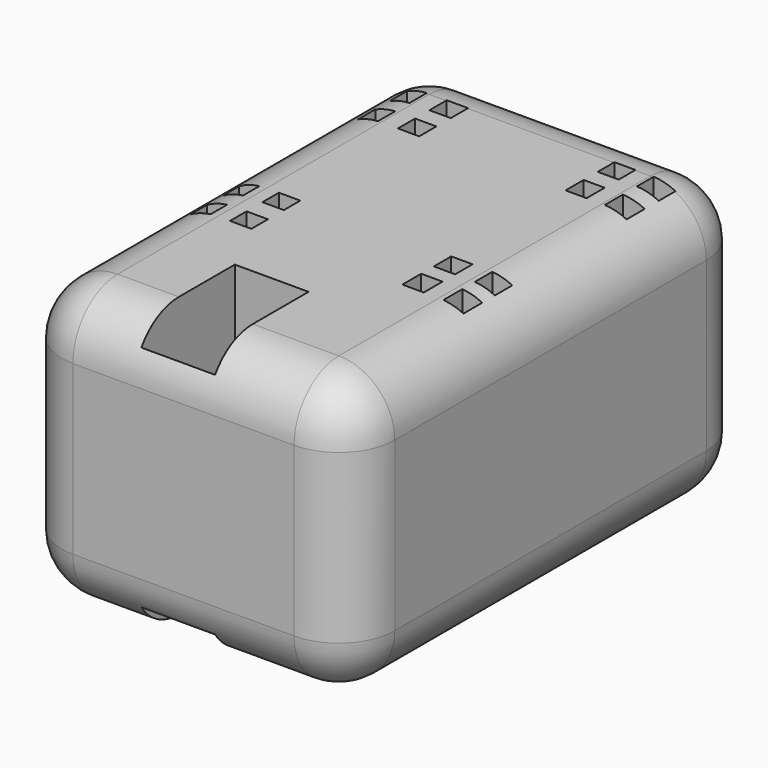
from build123d import *

# Parameters (mm, degrees)
F0_W         = 6.5923197919
F0_H         = 0.8001455572
F0_W_2       = 1.763837412
F0_H_2       = 1.412447542
F0_H_3       = 2.101770214
F0_W_3       = 1.9069323985
F0_H_4       = 1.9450464989
F0_W_4       = 1.7884944444
F0_W_5       = 1.6274210066
F0_H_5       = 1.5719905496
F0_H_6       = 1.8685259757
F0_W_6       = 1.9532360649
F0_H_7       = 2.0187458968
F0_W_7       = 1.8786090163
F0_W_8       = 1.7776318862
F0_H_8       = 1.6108304262
F0_W_9       = 1.7758645117
F0_H_9       = 1.9326903758
F0_H_10      = 1.91574162
F0_W_10      = 1.905767857
F0_W_11      = 1.7302669585
F0_H_11      = 1.8497077592
F0_H_12      = 1.7764922231
F0_H_13      = 1.8330642725
F0_W_12      = 1.8128681632
F0_W_13      = 1.9161291332
F1_DEPTH     = 25
F2_T1_DEPTH  = 34.8057161443
F2_T3_DEPTH  = 15
F2_T5_DEPTH  = 19.7681800186
F2_S9_W      = 5
F2_S9_H      = 5
F2_T10_DEPTH = 5
F2_S15_W     = 5
F2_S15_H     = 5
F2_T16_DEPTH = 5
F2_S21_W     = 5
F2_S21_H     = 5
F2_T22_DEPTH = 5
F2_S27_W     = 5
F2_S27_H     = 5
F2_T28_DEPTH = 5
F2_S33_W     = 5
F2_S33_H     = 5
F2_T34_DEPTH = 5
F2_S39_W     = 5
F2_S39_H     = 5
F2_T40_DEPTH = 5
F2_S45_W     = 5
F2_S45_H     = 5
F2_T46_DEPTH = 5
F2_S51_W     = 5
F2_S51_H     = 5
F2_T52_DEPTH = 5


# Not quite as in the source:
# - a fillet or chamfer that OpenCascade refuses, or shapes differently, is made with other operations: its cross-section is extruded or revolved along the edge and cut away or added


with BuildPart() as f1:
    # F0 (on Top) → F1 (new body)
    with BuildSketch(Plane.XY):
        with Locations((-41.465645377, 0.4000727786)):
            Rectangle(F0_W, F0_H)
        Polygon((-25.4717437439, 44.8057161443), (-55.2399237625, 44.8057161443), (-55.2399237625, 0), (-44.761805273, 0), (-44.761805273, 0.8001455572), (-44.761805273, 11.2422176864), (-38.1694854811, 11.2422176864), (-38.1694854811, 0.8001455572), (-38.1694854811, 0), (-25.4717437439, 0), (-25.4717437439, 44.1919353443), align=None)
        Polygon((-52.6931885334, 19.8126584291), (-52.6931885334, 21.6457227017), (-50.8803203702, 21.6457227017), (-49.1500534117, 21.6457227017), (-47.2339242785, 21.6457227017), (-47.2339242785, 19.8126584291), (-47.2339242785, 18.036166206), (-47.2339242785, 16.1864584468), (-49.1500534117, 16.1864584468), (-50.8803203702, 16.1864584468), (-52.6931885334, 16.1864584468), (-52.6931885334, 18.036166206), align=None, mode=Mode.SUBTRACT)
        Polygon((-30.0695020705, 21.6457227017), (-28.2810076261, 21.6457227017), (-28.2810076261, 19.7006762028), (-28.2810076261, 18.2882286608), (-28.2810076261, 16.1864584468), (-30.0695020705, 16.1864584468), (-31.8333394825, 16.1864584468), (-33.740271881, 16.1864584468), (-33.740271881, 18.2882286608), (-33.740271881, 19.7006762028), (-33.740271881, 21.6457227017), (-31.8333394825, 21.6457227017), align=None, mode=Mode.SUBTRACT)
        Polygon((-52.2811726703, 37.9449166358), (-52.2811726703, 39.8776070116), (-50.5035407841, 39.8776070116), (-48.7276762724, 39.8776070116), (-46.8219084154, 39.8776070116), (-46.8219084154, 37.9449166358), (-46.8219084154, 36.3340862095), (-46.8219084154, 34.4183445895), (-48.7276762724, 34.4183445895), (-50.5035407841, 34.4183445895), (-52.2811726703, 34.4183445895), (-52.2811726703, 36.3340862095), align=None, mode=Mode.SUBTRACT)
        Polygon((-30.2342418581, 39.8776070116), (-28.2810057933, 39.8776070116), (-28.2810057933, 38.0090810359), (-28.2810057933, 36.4370904863), (-28.2810057933, 34.4183445895), (-30.2342418581, 34.4183445895), (-31.8616628647, 34.4183445895), (-33.740271881, 34.4183445895), (-33.740271881, 36.4370904863), (-33.740271881, 38.0090810359), (-33.740271881, 39.8776070116), (-31.8616628647, 39.8776070116), align=None, mode=Mode.SUBTRACT)
        with Locations((-30.9514207765, 18.9944524318)):
            Rectangle(F0_W_2, F0_H_2)
        with Locations((-30.9514207765, 17.2373435538)):
            Rectangle(F0_W_2, F0_H_3)
        with Locations((-32.7868056818, 18.9944524318)):
            Rectangle(F0_W_3, F0_H_2)
        with Locations((-30.9514207765, 20.6731994522)):
            Rectangle(F0_W_2, F0_H_4)
        with Locations((-29.1752548483, 18.9944524318)):
            Rectangle(F0_W_4, F0_H_2)
        with Locations((-31.0479523614, 37.2230857611)):
            Rectangle(F0_W_5, F0_H_5)
        with Locations((-31.0479523614, 38.9433440237)):
            Rectangle(F0_W_5, F0_H_6)
        with Locations((-29.2576238257, 37.2230857611)):
            Rectangle(F0_W_6, F0_H_5)
        with Locations((-31.0479523614, 35.4277175379)):
            Rectangle(F0_W_5, F0_H_7)
        with Locations((-32.8009673728, 37.2230857611)):
            Rectangle(F0_W_7, F0_H_5)
        with Locations((-51.3923567272, 37.1395014226)):
            Rectangle(F0_W_8, F0_H_8)
        with Locations((-49.6156085283, 37.1395014226)):
            Rectangle(F0_W_9, F0_H_8)
        with Locations((-49.6156085283, 38.9112618237)):
            Rectangle(F0_W_9, F0_H_9)
        with Locations((-49.6156085283, 35.3762153995)):
            Rectangle(F0_W_9, F0_H_10)
        with Locations((-47.7747923439, 37.1395014226)):
            Rectangle(F0_W_10, F0_H_8)
        with Locations((-50.015186891, 17.1113123264)):
            Rectangle(F0_W_11, F0_H_11)
        with Locations((-50.015186891, 18.9244123176)):
            Rectangle(F0_W_11, F0_H_12)
        with Locations((-50.015186891, 20.7291905654)):
            Rectangle(F0_W_11, F0_H_13)
        with Locations((-51.7867544518, 18.9244123176)):
            Rectangle(F0_W_12, F0_H_12)
        with Locations((-48.1919888451, 18.9244123176)):
            Rectangle(F0_W_13, F0_H_12)
    extrude(amount=F1_DEPTH)

    # F2: fillet of radius 5 on 12 edges, made by hand

    # F2_s2 → F2_t1 (cut)
    with BuildSketch(Plane.XZ.offset(-39.8057161443)):
        with BuildLine():
            ThreePointArc((-25.4717437439, 5), (-26.9362098379, 1.4644660941), (-30.4717437439, 0))
            Line((-30.4717437439, 0), (-25.4717437439, 0))
            Line((-25.4717437439, 0), (-25.4717437439, 5))
        make_face()
        with BuildLine():
            ThreePointArc((-25.4717437439, 20), (-26.9362098379, 23.5355339059), (-30.4717437439, 25))
            Line((-30.4717437439, 25), (-25.4717437439, 25))
            Line((-25.4717437439, 25), (-25.4717437439, 20))
        make_face()
        with BuildLine():
            ThreePointArc((-55.2399237625, 5), (-53.7754576684, 1.4644660941), (-50.2399237625, 0))
            Line((-50.2399237625, 0), (-55.2399237625, 0))
            Line((-55.2399237625, 0), (-55.2399237625, 5))
        make_face()
        with BuildLine():
            ThreePointArc((-55.2399237625, 20), (-53.7754576684, 23.5355339059), (-50.2399237625, 25))
            Line((-50.2399237625, 25), (-55.2399237625, 25))
            Line((-55.2399237625, 25), (-55.2399237625, 20))
        make_face()
    extrude(amount=F2_T1_DEPTH, mode=Mode.SUBTRACT)

    # F2_s4 → F2_t3 (cut)
    with BuildSketch(Plane.XY.offset(5)):
        with BuildLine():
            ThreePointArc((-25.4717437439, 39.8057161443), (-26.9362098379, 43.3412500502), (-30.4717437439, 44.8057161443))
            Line((-30.4717437439, 44.8057161443), (-25.4717437439, 44.8057161443))
            Line((-25.4717437439, 44.8057161443), (-25.4717437439, 39.8057161443))
        make_face()
        with BuildLine():
            ThreePointArc((-50.2399237625, 44.8057161443), (-53.7754576684, 43.3412500502), (-55.2399237625, 39.8057161443))
            Line((-55.2399237625, 39.8057161443), (-55.2399237625, 44.8057161443))
            Line((-55.2399237625, 44.8057161443), (-50.2399237625, 44.8057161443))
        make_face()
        with BuildLine():
            ThreePointArc((-55.2399237625, 5), (-53.7754576684, 1.4644660941), (-50.2399237625, 0))
            Line((-50.2399237625, 0), (-55.2399237625, 0))
            Line((-55.2399237625, 0), (-55.2399237625, 5))
        make_face()
        with BuildLine():
            ThreePointArc((-25.4717437439, 5), (-26.9362098379, 1.4644660941), (-30.4717437439, 0))
            Line((-30.4717437439, 0), (-25.4717437439, 0))
            Line((-25.4717437439, 0), (-25.4717437439, 5))
        make_face()
    extrude(amount=F2_T3_DEPTH, mode=Mode.SUBTRACT)

    # F2_s6 → F2_t5 (cut)
    with BuildSketch(Plane.YZ.offset(-50.2399237625)):
        with BuildLine():
            ThreePointArc((44.8057161443, 5), (43.3412500502, 1.4644660941), (39.8057161443, 0))
            Line((39.8057161443, 0), (44.8057161443, 0))
            Line((44.8057161443, 0), (44.8057161443, 5))
        make_face()
        with BuildLine():
            ThreePointArc((44.8057161443, 20), (43.3412500502, 23.5355339059), (39.8057161443, 25))
            Line((39.8057161443, 25), (44.8057161443, 25))
            Line((44.8057161443, 25), (44.8057161443, 20))
        make_face()
        with BuildLine():
            ThreePointArc((0, 20), (1.4644660941, 23.5355339059), (5, 25))
            Line((5, 25), (0, 25))
            Line((0, 25), (0, 20))
        make_face()
        with BuildLine():
            ThreePointArc((0, 5), (1.4644660941, 1.4644660941), (5, 0))
            Line((5, 0), (0, 0))
            Line((0, 0), (0, 5))
        make_face()
    extrude(amount=F2_T5_DEPTH, mode=Mode.SUBTRACT)


with BuildPart() as f2_tool8:
    # F2_s9 → F2_t10 (new body)
    with BuildSketch(Plane.XY.offset(5)):
        with Locations((-27.9717437439, 2.5)):
            Rectangle(F2_S9_W, F2_S9_H)
    extrude(amount=-F2_T10_DEPTH)

    # F2_s11 → F2_t12 (revolve, cut)
    with BuildSketch(Plane(origin=(-30.4717437439, 5, 5), x_dir=(-0.7071067812, 0.7071067812, 0), z_dir=(-0.7071067812, -0.7071067812, 0))):
        with BuildLine():
            ThreePointArc((0, -5), (5, 0), (0, 5))
            Line((0, 5), (0, -5))
        make_face()
    revolve(axis=Axis((-30.4717437439, 5, 5), (0, 0, -1)), mode=Mode.SUBTRACT)


with BuildPart() as f1_1:
    add(f1.part)

    # F2_t7: cut F2_tool8
    add(f2_tool8.part, mode=Mode.SUBTRACT)


with BuildPart() as f2_tool14:
    # F2_s15 → F2_t16 (new body)
    with BuildSketch(Plane.XY.offset(5)):
        with Locations((-27.9717437439, 42.3057161443)):
            Rectangle(F2_S15_W, F2_S15_H)
    extrude(amount=-F2_T16_DEPTH)

    # F2_s17 → F2_t18 (revolve, cut)
    with BuildSketch(Plane(origin=(-30.4717437439, 39.8057161443, 5), x_dir=(-0.7071067812, -0.7071067812, 0), z_dir=(0.7071067812, -0.7071067812, 0))):
        with BuildLine():
            ThreePointArc((0, -5), (5, 0), (0, 5))
            Line((0, 5), (0, -5))
        make_face()
    revolve(axis=Axis((-30.4717437439, 39.8057161443, 5), (0, 0, -1)), mode=Mode.SUBTRACT)


with BuildPart() as f1_2:
    add(f1_1.part)

    # F2_t13: cut F2_tool14
    add(f2_tool14.part, mode=Mode.SUBTRACT)


with BuildPart() as f2_tool20:
    # F2_s21 → F2_t22 (new body)
    with BuildSketch(Plane.XY.offset(20)):
        with Locations((-27.9717437439, 42.3057161443)):
            Rectangle(F2_S21_W, F2_S21_H)
    extrude(amount=F2_T22_DEPTH)

    # F2_s23 → F2_t24 (revolve, cut)
    with BuildSketch(Plane(origin=(-30.4717437439, 39.8057161443, 20), x_dir=(-0.7071067812, -0.7071067812, 0), z_dir=(-0.7071067812, 0.7071067812, 0))):
        with BuildLine():
            ThreePointArc((0, -5), (5, 0), (0, 5))
            Line((0, 5), (0, -5))
        make_face()
    revolve(axis=Axis((-30.4717437439, 39.8057161443, 20), (0, 0, 1)), mode=Mode.SUBTRACT)


with BuildPart() as f1_3:
    add(f1_2.part)

    # F2_t19: cut F2_tool20
    add(f2_tool20.part, mode=Mode.SUBTRACT)


with BuildPart() as f2_tool26:
    # F2_s27 → F2_t28 (new body)
    with BuildSketch(Plane.XY.offset(20)):
        with Locations((-27.9717437439, 2.5)):
            Rectangle(F2_S27_W, F2_S27_H)
    extrude(amount=F2_T28_DEPTH)

    # F2_s29 → F2_t30 (revolve, cut)
    with BuildSketch(Plane(origin=(-30.4717437439, 5, 20), x_dir=(-0.7071067812, 0.7071067812, 0), z_dir=(0.7071067812, 0.7071067812, 0))):
        with BuildLine():
            ThreePointArc((0, -5), (5, 0), (0, 5))
            Line((0, 5), (0, -5))
        make_face()
    revolve(axis=Axis((-30.4717437439, 5, 20), (0, 0, 1)), mode=Mode.SUBTRACT)


with BuildPart() as f1_4:
    add(f1_3.part)

    # F2_t25: cut F2_tool26
    add(f2_tool26.part, mode=Mode.SUBTRACT)


with BuildPart() as f2_tool32:
    # F2_s33 → F2_t34 (new body)
    with BuildSketch(Plane.XY.offset(5)):
        with Locations((-52.7399237625, 42.3057161443)):
            Rectangle(F2_S33_W, F2_S33_H)
    extrude(amount=-F2_T34_DEPTH)

    # F2_s35 → F2_t36 (revolve, cut)
    with BuildSketch(Plane(origin=(-50.2399237625, 39.8057161443, 5), x_dir=(0.7071067812, -0.7071067812, 0), z_dir=(0.7071067812, 0.7071067812, 0))):
        with BuildLine():
            ThreePointArc((0, -5), (5, 0), (0, 5))
            Line((0, 5), (0, -5))
        make_face()
    revolve(axis=Axis((-50.2399237625, 39.8057161443, 5), (0, 0, -1)), mode=Mode.SUBTRACT)


with BuildPart() as f1_5:
    add(f1_4.part)

    # F2_t31: cut F2_tool32
    add(f2_tool32.part, mode=Mode.SUBTRACT)


with BuildPart() as f2_tool38:
    # F2_s39 → F2_t40 (new body)
    with BuildSketch(Plane.XY.offset(5)):
        with Locations((-52.7399237625, 2.5)):
            Rectangle(F2_S39_W, F2_S39_H)
    extrude(amount=-F2_T40_DEPTH)

    # F2_s41 → F2_t42 (revolve, cut)
    with BuildSketch(Plane(origin=(-50.2399237625, 5, 5), x_dir=(0.7071067812, 0.7071067812, 0), z_dir=(-0.7071067812, 0.7071067812, 0))):
        with BuildLine():
            ThreePointArc((0, -5), (5, 0), (0, 5))
            Line((0, 5), (0, -5))
        make_face()
    revolve(axis=Axis((-50.2399237625, 5, 5), (0, 0, -1)), mode=Mode.SUBTRACT)


with BuildPart() as f1_6:
    add(f1_5.part)

    # F2_t37: cut F2_tool38
    add(f2_tool38.part, mode=Mode.SUBTRACT)


with BuildPart() as f2_tool44:
    # F2_s45 → F2_t46 (new body)
    with BuildSketch(Plane.XY.offset(20)):
        with Locations((-52.7399237625, 42.3057161443)):
            Rectangle(F2_S45_W, F2_S45_H)
    extrude(amount=F2_T46_DEPTH)

    # F2_s47 → F2_t48 (revolve, cut)
    with BuildSketch(Plane(origin=(-50.2399237625, 39.8057161443, 20), x_dir=(0.7071067812, -0.7071067812, 0), z_dir=(-0.7071067812, -0.7071067812, 0))):
        with BuildLine():
            ThreePointArc((0, -5), (5, 0), (0, 5))
            Line((0, 5), (0, -5))
        make_face()
    revolve(axis=Axis((-50.2399237625, 39.8057161443, 20), (0, 0, 1)), mode=Mode.SUBTRACT)


with BuildPart() as f1_7:
    add(f1_6.part)

    # F2_t43: cut F2_tool44
    add(f2_tool44.part, mode=Mode.SUBTRACT)


with BuildPart() as f2_tool50:
    # F2_s51 → F2_t52 (new body)
    with BuildSketch(Plane.XY.offset(20)):
        with Locations((-52.7399237625, 2.5)):
            Rectangle(F2_S51_W, F2_S51_H)
    extrude(amount=F2_T52_DEPTH)

    # F2_s53 → F2_t54 (revolve, cut)
    with BuildSketch(Plane(origin=(-50.2399237625, 5, 20), x_dir=(0.7071067812, 0.7071067812, 0), z_dir=(0.7071067812, -0.7071067812, 0))):
        with BuildLine():
            ThreePointArc((0, -5), (5, 0), (0, 5))
            Line((0, 5), (0, -5))
        make_face()
    revolve(axis=Axis((-50.2399237625, 5, 20), (0, 0, 1)), mode=Mode.SUBTRACT)


with BuildPart() as f1_8:
    add(f1_7.part)

    # F2_t49: cut F2_tool50
    add(f2_tool50.part, mode=Mode.SUBTRACT)


solid = f1_8.part
